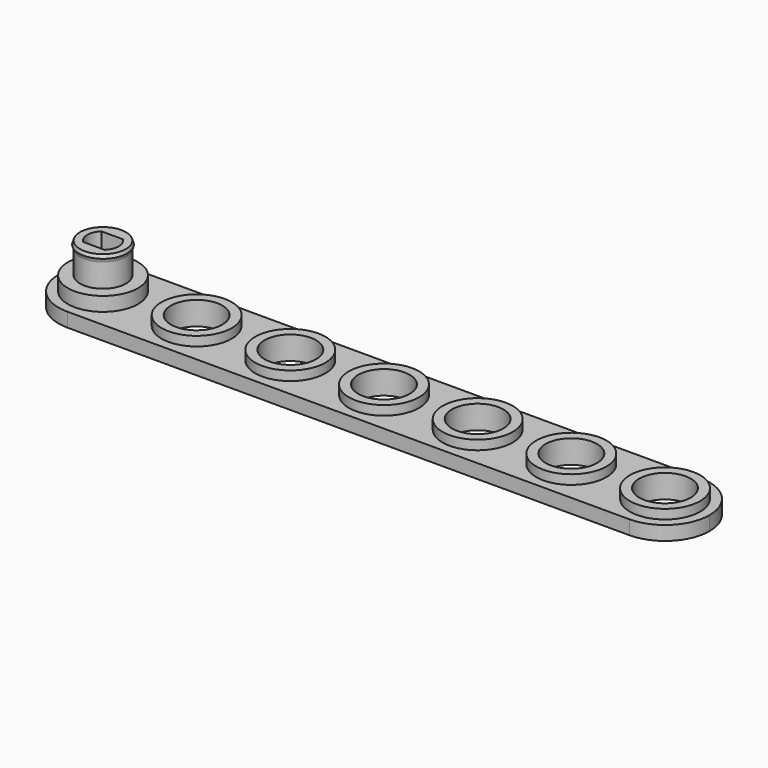
from build123d import *

# Parameters (mm, degrees)
F2_R     = 7.5
F2_R_2   = 5.5
F3_DEPTH = 3
F4_DEPTH = 5
F5_DEPTH = 5
F2_R_3   = 4.9
F6_DEPTH = 6
F7_DEPTH = 12.5


# Not quite as in the source:
# - a feature names something its author has since deleted; it is built from what else it names


with BuildPart() as f3:
    # F2 (on Top) → F3 (new body)
    with BuildSketch(Plane.XY):
        with BuildLine():
            Line((140, 9.5), (20, 9.5))
            ThreePointArc((20, 9.5), (10.5, 0), (20, -9.5))
            Line((20, -9.5), (140, -9.5))
            ThreePointArc((140, -9.5), (146.7175144213, -6.7175144213), (149.5, 0))
            ThreePointArc((149.5, 0), (146.7175144213, 6.7175144213), (140, 9.5))
        make_face()
        with Locations((20, 0)):
            Circle(F2_R, mode=Mode.SUBTRACT)
        with Locations((40, 0)):
            Circle(F2_R, mode=Mode.SUBTRACT)
        with Locations((60, 0)):
            Circle(F2_R, mode=Mode.SUBTRACT)
        with Locations((80, 0)):
            Circle(F2_R, mode=Mode.SUBTRACT)
        with Locations((100, 0)):
            Circle(F2_R, mode=Mode.SUBTRACT)
        with Locations((120, 0)):
            Circle(F2_R, mode=Mode.SUBTRACT)
        with Locations((140, 0)):
            Circle(F2_R, mode=Mode.SUBTRACT)
        with Locations((20, 0)):
            Circle(F2_R)
        with Locations((20, 0)):
            Circle(F2_R_2, mode=Mode.SUBTRACT)
        with Locations((40, 0)):
            Circle(F2_R)
        with Locations((40, 0)):
            Circle(F2_R_2, mode=Mode.SUBTRACT)
        with Locations((60, 0)):
            Circle(F2_R)
        with Locations((60, 0)):
            Circle(F2_R_2, mode=Mode.SUBTRACT)
        with Locations((80, 0)):
            Circle(F2_R)
        with Locations((80, 0)):
            Circle(F2_R_2, mode=Mode.SUBTRACT)
        with Locations((100, 0)):
            Circle(F2_R)
        with Locations((100, 0)):
            Circle(F2_R_2, mode=Mode.SUBTRACT)
        with Locations((120, 0)):
            Circle(F2_R)
        with Locations((120, 0)):
            Circle(F2_R_2, mode=Mode.SUBTRACT)
        with Locations((140, 0)):
            Circle(F2_R)
        with Locations((140, 0)):
            Circle(F2_R_2, mode=Mode.SUBTRACT)
    extrude(amount=F3_DEPTH)

    # F2 (on Top) → F4 (join)
    with BuildSketch(Plane.XY):
        with Locations((20, 0)):
            Circle(F2_R)
        with Locations((20, 0)):
            Circle(F2_R_2, mode=Mode.SUBTRACT)
        with Locations((40, 0)):
            Circle(F2_R)
        with Locations((40, 0)):
            Circle(F2_R_2, mode=Mode.SUBTRACT)
        with Locations((60, 0)):
            Circle(F2_R)
        with Locations((60, 0)):
            Circle(F2_R_2, mode=Mode.SUBTRACT)
        with Locations((80, 0)):
            Circle(F2_R)
        with Locations((80, 0)):
            Circle(F2_R_2, mode=Mode.SUBTRACT)
        with Locations((100, 0)):
            Circle(F2_R)
        with Locations((100, 0)):
            Circle(F2_R_2, mode=Mode.SUBTRACT)
        with Locations((120, 0)):
            Circle(F2_R)
        with Locations((120, 0)):
            Circle(F2_R_2, mode=Mode.SUBTRACT)
        with Locations((140, 0)):
            Circle(F2_R)
        with Locations((140, 0)):
            Circle(F2_R_2, mode=Mode.SUBTRACT)
    extrude(amount=F4_DEPTH)

    # F2 (on Top) → F5 (join)
    with BuildSketch(Plane.XY):
        with Locations((140, 0)):
            Circle(F2_R)
        with Locations((140, 0)):
            Circle(F2_R_2, mode=Mode.SUBTRACT)
    extrude(amount=F5_DEPTH)

    # F2 (on Top) → F6 (join)
    with BuildSketch(Plane.XY):
        with Locations((20, 0)):
            Circle(F2_R)
        with Locations((20, 0)):
            Circle(F2_R_2, mode=Mode.SUBTRACT)
        with Locations((20, 0)):
            Circle(F2_R_2)
        with Locations((20, 0)):
            Circle(F2_R_3, mode=Mode.SUBTRACT)
    extrude(amount=F6_DEPTH)

    # F2 (on Top) → F7 (join)
    with BuildSketch(Plane.XY):
        with Locations((20, 0)):
            Circle(F2_R_3)
        with BuildLine():
            Line((22.2847319318, -2.45), (20, -2.45))
            Line((20, -2.45), (17.7152680682, -2.45))
            ThreePointArc((17.7152680682, -2.45), (16.65, 0), (17.7152680682, 2.45))
            Line((17.7152680682, 2.45), (20, 2.45))
            Line((20, 2.45), (22.2847319318, 2.45))
            ThreePointArc((22.2847319318, 2.45), (23.35, 0), (22.2847319318, -2.45))
        make_face(mode=Mode.SUBTRACT)
    extrude(amount=F7_DEPTH)

    # F9 (on plane+point) → F10 (revolve)
    with BuildSketch(Plane.XZ):
        Polygon((25.15, 11.75), (24.9, 12.5), (24.9, 11), align=None)
    revolve(axis=Axis((20, 0, 6.25), (0, 0, 1)))


solid = f3.part
